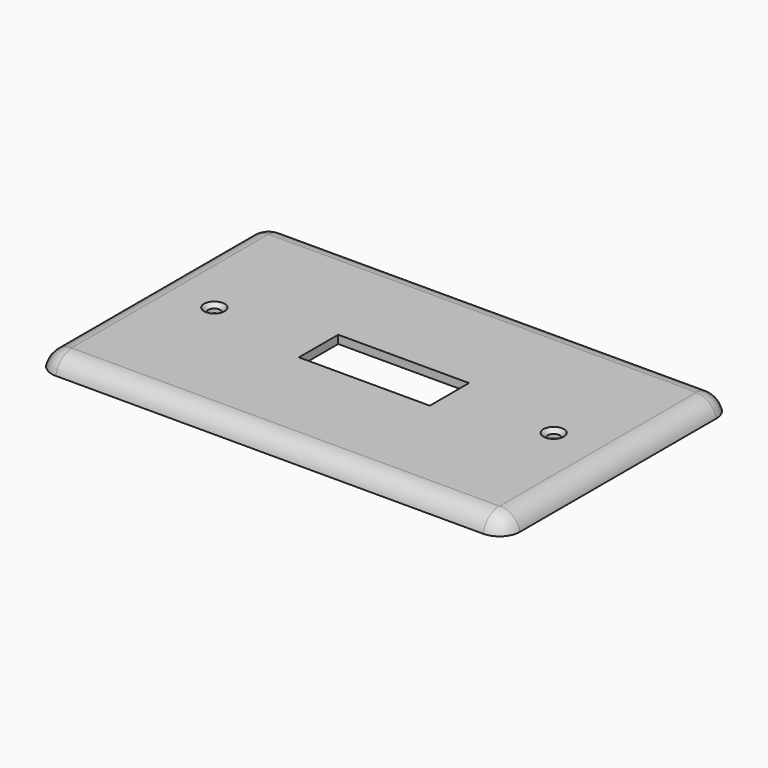
from build123d import *

# Parameters (mm, degrees)
F0_W           = 114.5
F0_H           = 70
F1_DEPTH       = 4
F2_R           = 5
F3_T1_DEPTH    = 104.5
F3_T3_DEPTH    = 60
F3_T6_ANGLE    = 90
F3_T8_ANGLE    = 90
F3_T10_ANGLE   = 90
F3_T12_ANGLE   = 90
F4_T           = -2
F5_W           = 32
F5_H           = 12
F6_DEPTH       = 4.0010001078
F8_D           = 3
F8_CSINK_D     = 5
F8_CSINK_ANGLE = 90


# Not quite as in the source:
# - a fillet or chamfer that OpenCascade refuses, or shapes differently, is made with other operations: its cross-section is extruded or revolved along the edge and cut away or added


with BuildPart() as f1:
    # F0 (on Top) → F1 (new body)
    with BuildSketch(Plane.XY):
        Rectangle(F0_W, F0_H)
    extrude(amount=F1_DEPTH)

    # F2
    f2_edges = [f1.edges().sort_by_distance(p)[0] for p in [
        (-57.25, 35, 2),
        (57.25, 35, 2),
        (-57.25, -35, 2),
        (57.25, -35, 2),
    ]]
    fillet(f2_edges, radius=F2_R)

    # F3: fillet of radius 5 on 8 edges, made by hand

    # F3_s2 → F3_t1 (cut)
    with BuildSketch(Plane.YZ.offset(-52.25)):
        with BuildLine():
            ThreePointArc((-30.1010205144, 4), (-33.2632981746, 2.8729833462), (-35, 0))
            Line((-35, 0), (-35, 4))
            Line((-35, 4), (-30.1010205144, 4))
        make_face()
        with BuildLine():
            ThreePointArc((35, 0), (33.2632981746, 2.8729833462), (30.1010205144, 4))
            Line((30.1010205144, 4), (35, 4))
            Line((35, 4), (35, 0))
        make_face()
    extrude(amount=F3_T1_DEPTH, mode=Mode.SUBTRACT)

    # F3_s4 → F3_t3 (cut)
    with BuildSketch(Plane.XZ.offset(-30)):
        with BuildLine():
            ThreePointArc((-52.3510205144, 4), (-55.5132981746, 2.8729833462), (-57.25, 0))
            Line((-57.25, 0), (-57.25, 4))
            Line((-57.25, 4), (-52.3510205144, 4))
        make_face()
        with BuildLine():
            ThreePointArc((52.3510205144, 4), (55.5132981746, 2.8729833462), (57.25, 0))
            Line((57.25, 0), (57.25, 4))
            Line((57.25, 4), (52.3510205144, 4))
        make_face()
    extrude(amount=F3_T3_DEPTH, mode=Mode.SUBTRACT)

    # F3_s5 → F3_t6 (revolve, cut)
    with BuildSketch(Plane.XZ.offset(30)):
        with BuildLine():
            ThreePointArc((-52.3510205144, 4), (-55.5132981746, 2.8729833462), (-57.25, 0))
            Line((-57.25, 0), (-57.25, 4))
            Line((-57.25, 4), (-52.3510205144, 4))
        make_face()
    revolve(axis=Axis((-52.25, -30, 4), (0, 0, 1)), revolution_arc=F3_T6_ANGLE, mode=Mode.SUBTRACT)

    # F3_s7 → F3_t8 (revolve, cut)
    with BuildSketch(Plane.YZ.offset(52.25)):
        with BuildLine():
            ThreePointArc((-30.1010205144, 4), (-33.2632981746, 2.8729833462), (-35, 0))
            Line((-35, 0), (-35, 4))
            Line((-35, 4), (-30.1010205144, 4))
        make_face()
    revolve(axis=Axis((52.25, -30, 4), (0, 0, 1)), revolution_arc=F3_T8_ANGLE, mode=Mode.SUBTRACT)

    # F3_s9 → F3_t10 (revolve, cut)
    with BuildSketch(Plane.YZ.offset(52.25)):
        with BuildLine():
            ThreePointArc((35, 0), (33.2632981746, 2.8729833462), (30.1010205144, 4))
            Line((30.1010205144, 4), (35, 4))
            Line((35, 4), (35, 0))
        make_face()
    revolve(axis=Axis((52.25, 30, 4), (0, 0, -1)), revolution_arc=F3_T10_ANGLE, mode=Mode.SUBTRACT)

    # F3_s11 → F3_t12 (revolve, cut)
    with BuildSketch(Plane.YZ.offset(-52.25)):
        with BuildLine():
            ThreePointArc((35, 0), (33.2632981746, 2.8729833462), (30.1010205144, 4))
            Line((30.1010205144, 4), (35, 4))
            Line((35, 4), (35, 0))
        make_face()
    revolve(axis=Axis((-52.25, 30, 4), (0, 0, 1)), revolution_arc=F3_T12_ANGLE, mode=Mode.SUBTRACT)

    # F4
    f4_openings = [f1.faces().sort_by_distance(p)[0] for p in [
        (0, 0, 0),
    ]]
    offset(amount=F4_T, openings=f4_openings)

    # F5 (on face) → F6 (cut, through all)
    with BuildSketch(Plane.XY.offset(4)):
        Rectangle(F5_W, F5_H)
    extrude(amount=-F6_DEPTH, mode=Mode.SUBTRACT)

    # F8 (through all)
    with Locations(Plane.XY.offset(4)):
        with Locations((41.5, 0), (-41.5, 0)):
            CounterSinkHole(F8_D / 2, F8_CSINK_D / 2, counter_sink_angle=F8_CSINK_ANGLE)


solid = f1.part
